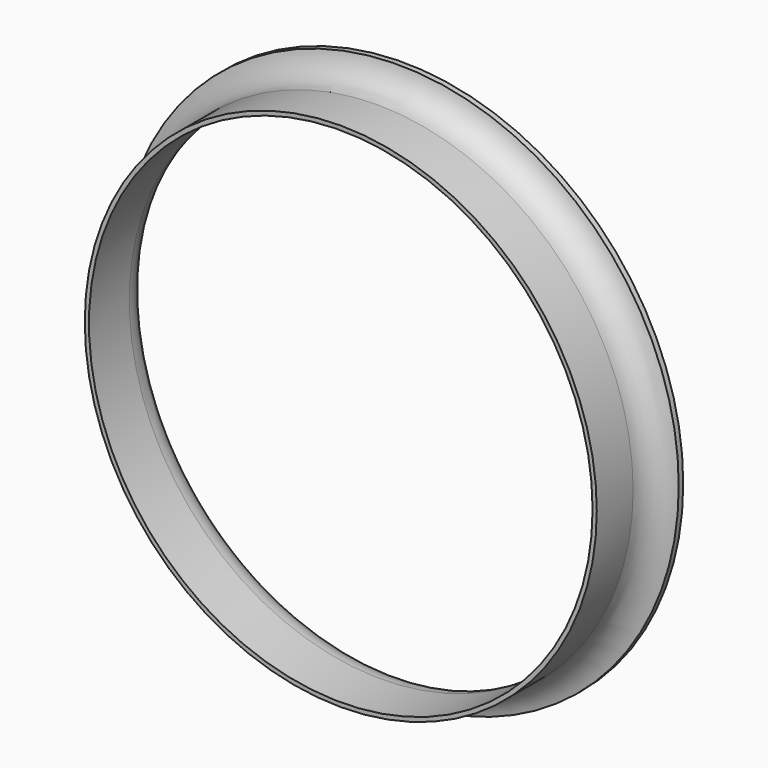
from build123d import *

# Parameters (mm, degrees)
F0_R     = 50
F0_R_2   = 45
F1_DEPTH = 1
F2_R     = 45.75
F3_DEPTH = 14
F5_R     = 45
F6_DEPTH = 17
F7_R     = 4.99999


# Not quite as in the source:
# - a fillet or chamfer that OpenCascade refuses, or shapes differently, is made with other operations: its cross-section is extruded or revolved along the edge and cut away or added
# - a fillet or chamfer is up to 0.001 mm smaller than in the source, because OpenCascade refuses the exact size


with BuildPart() as f1:
    # F0 (on Front) → F1 (new body)
    with BuildSketch(Plane.XZ):
        Circle(F0_R)
        Circle(F0_R_2, mode=Mode.SUBTRACT)
    extrude(amount=F1_DEPTH)

    # F2 (on Front) → F3 (join)
    with BuildSketch(Plane.XZ):
        Circle(F2_R)
    extrude(amount=F3_DEPTH)

    # F4: fillet of radius 5 on 1 edges, made by hand

    # F4_s1 → F4_t2 (revolve)
    with BuildSketch(Plane.XY):
        with BuildLine():
            ThreePointArc((49.9999399343, -0.9996045356), (46.9582217487, -2.6840834341), (45.7496, -5.9442601394))
            Line((45.7496, -5.9442601394), (45.2494634315, -5.9442601394))
            ThreePointArc((45.2494634315, -5.9442601394), (45.2498634315, -3.4721300697), (45.2498634315, -1))
            Line((45.2498634315, -1), (45.75, -0.4998634315))
            ThreePointArc((45.75, -0.4998634315), (47.8749699672, -0.4998634315), (49.9248373592, -0.5051389752))
            Line((49.9248373592, -0.5051389752), (49.9999399343, -0.9996045356))
        make_face()
    revolve(axis=Axis((0, -1, 0), (0, 1, 0)))

    # F5 (on face) → F6 (cut)
    with BuildSketch(Plane.XZ.offset(14)):
        Circle(F5_R)
    extrude(amount=-F6_DEPTH, mode=Mode.SUBTRACT)

    # F7 (radius 5 in the source; OpenCascade refuses exactly that, so slightly less here)
    f7_edges = [f1.edges().sort_by_distance(p)[0] for p in [
        (-45, 0, 0),
    ]]
    fillet(f7_edges, radius=F7_R)


solid = f1.part
